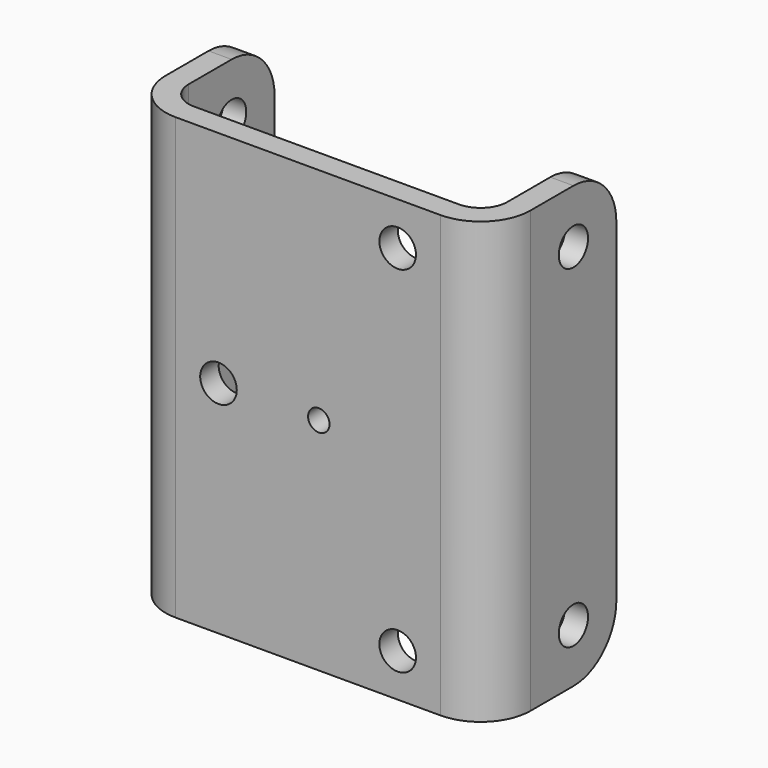
from build123d import *

# Parameters (mm, degrees)
F1_DEPTH = 32.5777606
F2_R     = 3.69316
F3_R     = 1.98374
F4_R     = 1.35255
F5_DEPTH = 26.9875
F6_R     = 3.96875
F7_R     = 0.79375
F7_R_2   = 1.35255
F8_DEPTH = 1.70942


with BuildPart() as f1:
    # F0 (on Top) → F1 (new body)
    with BuildSketch(Plane.XY):
        Polygon((0, 9.92124), (0, 0), (-23.56866, 0), (-23.56866, 9.92124), (-25.27808, 9.92124), (-25.27808, -1.70942), (1.70942, -1.70942), (1.70942, 9.92124), align=None)
    extrude(amount=F1_DEPTH)

    # F2
    f2_edges = [f1.edges().sort_by_distance(p)[0] for p in [
        (1.70942, -1.70942, 16.28888),
        (-25.27808, -1.70942, 16.28888),
    ]]
    fillet(f2_edges, radius=F2_R)

    # F3
    f3_edges = [f1.edges().sort_by_distance(p)[0] for p in [
        (0, 0, 16.28888),
        (-23.56866, 0, 16.28888),
    ]]
    fillet(f3_edges, radius=F3_R)

    # F4 (on face) → F5 (cut, through all)
    with BuildSketch(Plane.YZ.offset(1.70942)):
        with Locations((5.95249, 3.96875)):
            Circle(F4_R)
        with Locations((5.95249, 28.6090106)):
            Circle(F4_R)
    extrude(amount=-F5_DEPTH, mode=Mode.SUBTRACT)

    # F6
    f6_edges = [f1.edges().sort_by_distance(p)[0] for p in [
        (0.85471, 9.92124, 32.577761),
        (-24.42337, 9.92124, 32.577761),
        (0.85471, 9.92124, 0),
        (-24.42337, 9.92124, 0),
    ]]
    fillet(f6_edges, radius=F6_R)

    # F7 (on face) → F8 (cut, through all)
    with BuildSketch(Plane.XZ.offset(1.70942)):
        with Locations((-10.99058, 16.2888803)):
            Circle(F7_R)
        with Locations((-18.40992, 16.2888803)):
            Circle(F7_R_2)
        with Locations((-5.15874, 29.4027606)):
            Circle(F7_R_2)
        with Locations((-5.15874, 3.175)):
            Circle(F7_R_2)
    extrude(amount=-F8_DEPTH, mode=Mode.SUBTRACT)


solid = f1.part
